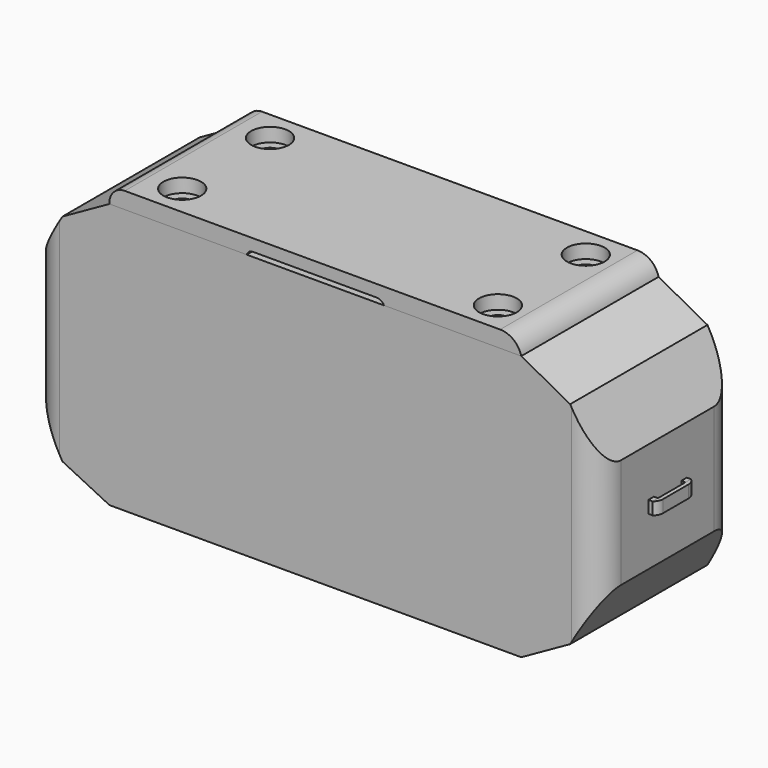
from build123d import *

# Parameters (mm, degrees)
F1_DEPTH       = 15.875
F2_DEPTH       = 15.875
F3_DEPTH       = 13.716
F4_R           = 3.4925
F4_R_2         = 1.8415
F5_DEPTH       = 2.54
F6_DEPTH       = 2.794
F7_W           = 1.27
F7_H           = 1.143
F8_DEPTH       = 0.762
F9_W           = 8.89
F9_H           = 2.286
F10_DEPTH      = 0.762
F11_R          = 5.08
F14_DEPTH      = 0.762
F15_W          = 8.89
F15_H          = 2.286
F16_DEPTH      = 0.762
F17_T1_DEPTH   = 9.5815945611
F17_2_T1_DEPTH = 9.5815945611


# Not quite as in the source:
# - a fillet or chamfer that OpenCascade refuses, or shapes differently, is made with other operations: its cross-section is extruded or revolved along the edge and cut away or added
# - a feature names something its author has since deleted; it is built from what else it names


with BuildPart() as f1:
    # F0 (on Front) → F1 (new body, symmetric)
    with BuildSketch(Plane.XZ):
        Polygon((-52.4684097937, 14.3684097937), (-38.1, 0), (0, 0), (38.1, 0), (52.4684097937, 14.3684097937), (52.4684097937, 34.6884097937), (38.1, 49.0568195874), (12.7, 49.0568195874), (-12.7, 49.0568195874), (-38.1, 49.0568195874), (-52.4684097937, 34.6884097937), align=None)
        Polygon((-46.8117259443, 4.2893581497), (-38.1, 0), (-52.4684097937, 14.3684097937), align=None)
        Polygon((-46.8117259443, 44.167522341), (-52.4684097937, 34.6884097937), (-38.1, 49.0568195874), align=None)
        Polygon((38.1, 49.0568195874), (52.4684097937, 34.6884097937), (47.1484308168, 44.167522341), align=None)
        Polygon((52.4684097937, 14.3684097937), (38.1, 0), (47.1484308168, 5.0782667132), align=None)
    extrude(amount=F1_DEPTH, both=True)

    # F11
    f11_edges = [f1.edges().sort_by_distance(p)[0] for p in [
        (-52.46841, -15.875, 24.52841),
        (-52.46841, 15.875, 24.52841),
        (52.46841, -15.875, 24.52841),
        (52.46841, 15.875, 24.52841),
    ]]
    fillet(f11_edges, radius=F11_R)


with BuildPart() as f2:
    # F0 (on Front) → F2 (new body, symmetric)
    with BuildSketch(Plane.XZ):
        with BuildLine():
            ThreePointArc((-35.2670811117, 52.1118827164), (-37.3502781829, 51.2026079726), (-38.1, 49.0568195874))
            Line((-38.1, 49.0568195874), (-12.7, 49.0568195874))
            ThreePointArc((-12.7, 49.0568195874), (-12.275793737, 49.6626248219), (-11.5737691522, 49.8952455819))
            Line((-11.5737691522, 49.8952455819), (11.3571360707, 49.8952455819))
            ThreePointArc((11.3571360707, 49.8952455819), (12.1486917669, 49.6684286067), (12.7, 49.0568195874))
            Line((12.7, 49.0568195874), (38.1, 49.0568195874))
            ThreePointArc((38.1, 49.0568195874), (36.6717162303, 51.25750972), (34.1911762953, 52.1118827164))
            Line((34.1911762953, 52.1118827164), (-35.2670811117, 52.1118827164))
        make_face()
    extrude(amount=F2_DEPTH, both=True)

    # F4 (on face) → F5 (cut)
    with BuildSketch(Plane.XY.offset(52.1118827164)):
        with Locations((29.21, -10.16)):
            Circle(F4_R)
        with Locations((29.21, -10.16)):
            Circle(F4_R_2, mode=Mode.SUBTRACT)
        with Locations((-29.21, -10.16)):
            Circle(F4_R)
        with Locations((-29.21, -10.16)):
            Circle(F4_R_2, mode=Mode.SUBTRACT)
        with Locations((-29.21, 10.16)):
            Circle(F4_R)
        with Locations((-29.21, 10.16)):
            Circle(F4_R_2, mode=Mode.SUBTRACT)
        with Locations((29.21, 10.16)):
            Circle(F4_R)
        with Locations((29.21, 10.16)):
            Circle(F4_R_2, mode=Mode.SUBTRACT)
    extrude(amount=-F5_DEPTH, mode=Mode.SUBTRACT)

    # F4 (on face) → F6 (cut)
    with BuildSketch(Plane.XY.offset(52.1118827164)):
        with Locations((-29.21, -10.16)):
            Circle(F4_R_2)
        with Locations((29.21, 10.16)):
            Circle(F4_R_2)
        with Locations((29.21, -10.16)):
            Circle(F4_R_2)
        with Locations((-29.21, 10.16)):
            Circle(F4_R_2)
    extrude(amount=-F6_DEPTH, mode=Mode.SUBTRACT)


with BuildPart() as f3:
    # F0 (on Front) → F3 (new body, symmetric)
    with BuildSketch(Plane.XZ):
        with BuildLine():
            ThreePointArc((-11.5737691522, 49.8952455819), (-12.275793737, 49.6626248219), (-12.7, 49.0568195874))
            Line((-12.7, 49.0568195874), (12.7, 49.0568195874))
            ThreePointArc((12.7, 49.0568195874), (12.1486917669, 49.6684286067), (11.3571360707, 49.8952455819))
            Line((11.3571360707, 49.8952455819), (-11.5737691522, 49.8952455819))
        make_face()
    extrude(amount=F3_DEPTH, both=True)


with BuildPart() as f8:
    # F7 (on face) → F8 (new body)
    with BuildSketch(Plane(origin=(-52.4684097937, 0, 0), x_dir=(0, -1, 0), z_dir=(-1, 0, 0))):
        with Locations((-3.81, 25.0999097937)):
            Rectangle(F7_W, F7_H)
        with Locations((-3.81, 23.9569097937)):
            Rectangle(F7_W, F7_H)
    extrude(amount=F8_DEPTH)


with BuildPart() as f8b:
    # F7 (on face) → F8, piece 2 (new body)
    with BuildSketch(Plane(origin=(-52.4684097937, 0, 0), x_dir=(0, -1, 0), z_dir=(-1, 0, 0))):
        with Locations((3.81, 25.0999097937)):
            Rectangle(F7_W, F7_H)
        with Locations((3.81, 23.9569097937)):
            Rectangle(F7_W, F7_H)
    extrude(amount=F8_DEPTH)


with BuildPart() as f10:
    # F9 (on face) → F10 (new body)
    with BuildSketch(Plane(origin=(-53.2304097937, 0, 0), x_dir=(0, -1, 0), z_dir=(-1, 0, 0))):
        with Locations((0, 24.5284097937)):
            Rectangle(F9_W, F9_H)
    extrude(amount=F10_DEPTH)

    # F17: fillet of radius 1.778 on 2 edges, made by hand

    # F17_s2 → F17_t1 (cut)
    with BuildSketch(Plane.XY.offset(19.7376125131)):
        with BuildLine():
            ThreePointArc((-53.2304097937, 4.445), (-53.7904383468, 3.8089351565), (-53.9924097937, 2.9858810878))
            Line((-53.9924097937, 2.9858810878), (-53.9924097937, 4.445))
            Line((-53.9924097937, 4.445), (-53.2304097937, 4.445))
        make_face()
        with BuildLine():
            ThreePointArc((-53.2304097937, -4.445), (-53.7904383468, -3.8089351565), (-53.9924097937, -2.9858810878))
            Line((-53.9924097937, -2.9858810878), (-53.9924097937, -4.445))
            Line((-53.9924097937, -4.445), (-53.2304097937, -4.445))
        make_face()
    extrude(amount=F17_T1_DEPTH, mode=Mode.SUBTRACT)


with BuildPart() as f14:
    # F13 (on face) → F14 (new body)
    with BuildSketch(Plane.YZ.offset(52.4684097937)):
        Polygon((-3.175, 23.3854097937), (-3.175, 24.5284097937), (-3.175, 25.6714097937), (-4.445, 25.6714097937), (-4.445, 23.3854097937), align=None)
    extrude(amount=F14_DEPTH)


with BuildPart() as f14b:
    # F13 (on face) → F14, piece 2 (new body)
    with BuildSketch(Plane.YZ.offset(52.4684097937)):
        Polygon((3.175, 25.6714097937), (3.175, 24.5284097937), (3.175, 23.3854097937), (4.445, 23.3854097937), (4.445, 25.6714097937), align=None)
    extrude(amount=F14_DEPTH)


with BuildPart() as f16:
    # F15 (on face) → F16 (new body)
    with BuildSketch(Plane.YZ.offset(53.2304097937)):
        with Locations((0, 24.5284097937)):
            Rectangle(F15_W, F15_H)
    extrude(amount=F16_DEPTH)

    # F17#2: fillet of radius 1.778 on 2 edges, made by hand

    # F17_2_s2 → F17_2_t1 (cut)
    with BuildSketch(Plane.XY.offset(19.7376125131)):
        with BuildLine():
            ThreePointArc((53.2304097937, -4.445), (53.7904383468, -3.8089351565), (53.9924097937, -2.9858810878))
            Line((53.9924097937, -2.9858810878), (53.9924097937, -4.445))
            Line((53.9924097937, -4.445), (53.2304097937, -4.445))
        make_face()
        with BuildLine():
            ThreePointArc((53.2304097937, 4.445), (53.7904383468, 3.8089351565), (53.9924097937, 2.9858810878))
            Line((53.9924097937, 2.9858810878), (53.9924097937, 4.445))
            Line((53.9924097937, 4.445), (53.2304097937, 4.445))
        make_face()
    extrude(amount=F17_2_T1_DEPTH, mode=Mode.SUBTRACT)


solid = Compound([f1.part, f2.part, f3.part, f8.part, f8b.part, f10.part, f14.part, f14b.part, f16.part])
